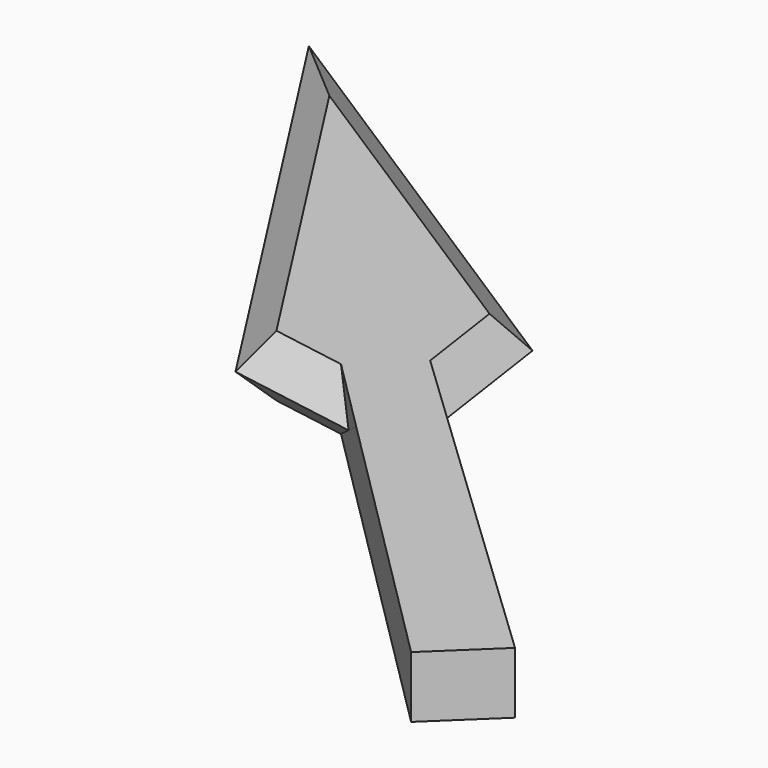
from build123d import *

# Parameters (mm, degrees)
F4_DEPTH     = 5.08
F5_SIZE2     = 5.07999
F5_SIZE      = 5.07999
F6_T1_DEPTH  = 83.8598569958
F6_T3_DEPTH  = 84.6306377444
F6_T8_DEPTH  = 42.5046669686
F6_T13_DEPTH = 41.8031738059


# Not quite as in the source:
# - a fillet or chamfer that OpenCascade refuses, or shapes differently, is made with other operations: its cross-section is extruded or revolved along the edge and cut away or added
# - a fillet or chamfer is up to 0.001 mm smaller than in the source, because OpenCascade refuses the exact size
# - the program builds the solid bodies; features that only make, move or delete a surface that nothing else refers to are left out


with BuildPart() as f4:
    # F0 (on Top) → F4 (new body)
    with BuildSketch(Plane.XY):
        Polygon((-2.3713386618, 16.203770414), (-51.0019175708, 47.3164618015), (-19.3783510476, -1.9021694316), (-3.9232242852, -4.51765256), (18.5309383262, -26.9124830378), (23.3981461688, -22.2631122398), (0, 0), align=None)
    extrude(amount=F4_DEPTH)

    # F5 (size 5.08 and 5.08 in the source; OpenCascade refuses exactly that, so slightly less here)
    f5_edges = [f4.edges().sort_by_distance(p)[0] for p in [
        (-11.650788, -3.209911, 0),
        (-35.190134, 22.707146, 0),
        (-26.686628, 31.760116, 0),
        (-1.185669, 8.101885, 0),
    ]]
    chamfer(f5_edges, length=F5_SIZE, length2=F5_SIZE2)

    # F6: chamfer of 5.08 on 4 edges, made by hand

    # F6_s2 → F6_t1 (cut)
    with BuildSketch(Plane(origin=(1.9661453214, -1.2578931606, 0), x_dir=(0, 0, 1), z_dir=(-0.8423569488, 0.5389200041, 0))):
        Polygon((0, 12.3713967634), (5.08, 7.2913967634), (5.08, 12.3713967634), align=None)
    extrude(amount=F6_T1_DEPTH, mode=Mode.SUBTRACT)

    # F6_s4 → F6_t3 (cut)
    with BuildSketch(Plane(origin=(-43.4826566064, 67.6760111474, 0), x_dir=(0, 0, 1), z_dir=(0.5405521777, -0.8413104915, 0))):
        Polygon((5.08, 12.2514318739), (0, 17.3314318739), (5.08, 17.3314318739), align=None)
    extrude(amount=F6_T3_DEPTH, mode=Mode.SUBTRACT)


with BuildPart() as f6_tool6:
    # F6_s7 → F6_t8 (new body)
    with BuildSketch(Plane(origin=(1.8917212496, -12.9264610367, 0), x_dir=(0, 0, 1), z_dir=(-0.1448024793, 0.9894605813, 0))):
        Polygon((0, 0), (5.08, -5.08), (5.08, 0), align=None)
    extrude(amount=F6_T8_DEPTH)

    split(bisect_by=Plane(origin=(0, 0, 0), x_dir=(0, 0, 1), z_dir=(0.6893167986, 0.7244600411, 0)), keep=Keep.TOP)


with BuildPart() as f4_1:
    add(f4.part)

    # F6_t5: cut F6_tool6
    add(f6_tool6.part, mode=Mode.SUBTRACT)


with BuildPart() as f6_tool11:
    # F6_s12 → F6_t13 (new body)
    with BuildSketch(Plane(origin=(-31.4068834176, 5.3150113201, 0), x_dir=(0, 0, 1), z_dir=(0.985980884, -0.1668583122, 0))):
        Polygon((5.08, 0.0289416476), (0, 5.1089416476), (5.08, 5.1089416476), align=None)
    extrude(amount=F6_T13_DEPTH)

    split(bisect_by=Plane(origin=(-4.2152403692, -4.2264080896, 0), x_dir=(0, 0, 1), z_dir=(-0.7061707096, -0.7080416152, 0)), keep=Keep.TOP)


with BuildPart() as f4_2:
    add(f4_1.part)

    # F6_t10: cut F6_tool11
    add(f6_tool11.part, mode=Mode.SUBTRACT)


solid = f4_2.part
